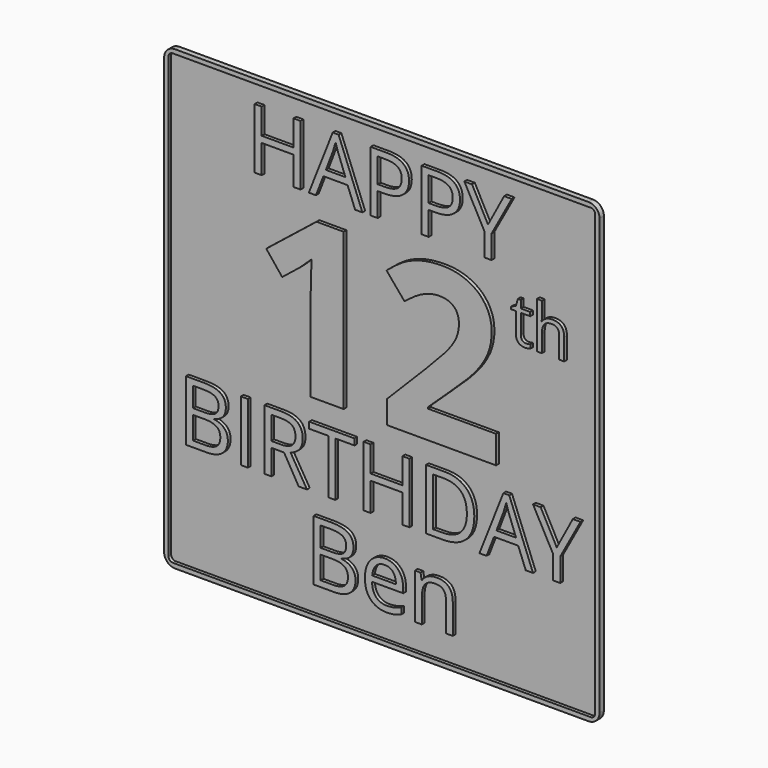
from build123d import *

# Parameters (mm, degrees)
F1_DEPTH       = 0.6
F2_TEXT_SIZE   = 24.6944444444
F2_TEXT_SIZE_2 = 63.7886434631
F2_TEXT_SIZE_3 = 17.7540454186
F3_DEPTH       = 1
F5_DEPTH       = 0.9906


# Not quite as in the source:
# - Text() gives the source's letters only with a copy of the font that has no kerning and outlines rounded to 1/6400 em; it was checked with that copy


with BuildPart() as f1:
    # F0 (on Front) → F1 (new body)
    with BuildSketch(Plane.XZ):
        with BuildLine():
            Line((123.825, 0), (3.175, 0))
            ThreePointArc((3.175, 0), (0.9299359697, -0.9299359697), (0, -3.175))
            Line((0, -3.175), (0, -130.175))
            ThreePointArc((0, -130.175), (0.9299359697, -132.4200640303), (3.175, -133.35))
            Line((3.175, -133.35), (123.825, -133.35))
            ThreePointArc((123.825, -133.35), (126.0700640303, -132.4200640303), (127, -130.175))
            Line((127, -130.175), (127, -3.175))
            ThreePointArc((127, -3.175), (126.0700640303, -0.9299359697), (123.825, 0))
        make_face()
    extrude(amount=F1_DEPTH)

    # F2 (on face) → F3 (join)
    with BuildSketch(Plane.XZ.offset(0.6)):
        with Locations((23.9946766493, -24.13)):
            Text('HAPPY', F2_TEXT_SIZE, font='Open Sans', text_align=(TextAlign.LEFT, TextAlign.BOTTOM))
        with Locations((3.9535915799, -100.5378232934)):
            Text('BIRTHDAY', F2_TEXT_SIZE, font='Open Sans', text_align=(TextAlign.LEFT, TextAlign.BOTTOM))
        with Locations((26.034138941, -76.4078232934)):
            Text('12', F2_TEXT_SIZE_2, font='Open Sans', font_style=FontStyle.BOLD, text_align=(TextAlign.LEFT, TextAlign.BOTTOM))
        with Locations((100.965861059, -43.2629127014)):
            Text('th', F2_TEXT_SIZE_3, font='Open Sans', text_align=(TextAlign.LEFT, TextAlign.BOTTOM))
        with Locations((41.1862543403, -124.3073880959)):
            Text('Ben', F2_TEXT_SIZE, font='Open Sans', text_align=(TextAlign.LEFT, TextAlign.BOTTOM))
    extrude(amount=F3_DEPTH)

    # F4 (on face) → F5 (join)
    with BuildSketch(Plane.XZ.offset(0.6)):
        with BuildLine():
            Line((127, -130.175), (127, -3.175))
            ThreePointArc((127, -3.175), (126.0700640303, -0.9299359697), (123.825, 0))
            Line((123.825, 0), (3.175, 0))
            ThreePointArc((3.175, 0), (0.9299359697, -0.9299359697), (0, -3.175))
            Line((0, -3.175), (0, -130.175))
            ThreePointArc((0, -130.175), (0.9299359697, -132.4200640303), (3.175, -133.35))
            Line((3.175, -133.35), (123.825, -133.35))
            ThreePointArc((123.825, -133.35), (126.0700640303, -132.4200640303), (127, -130.175))
        make_face()
        with BuildLine():
            ThreePointArc((1.27, -2.54), (1.6419743879, -1.6419743879), (2.54, -1.27))
            Line((2.54, -1.27), (124.46, -1.27))
            ThreePointArc((124.46, -1.27), (125.3580256121, -1.6419743879), (125.73, -2.54))
            Line((125.73, -2.54), (125.73, -130.81))
            ThreePointArc((125.73, -130.81), (125.3580256121, -131.7080256121), (124.46, -132.08))
            Line((124.46, -132.08), (2.54, -132.08))
            ThreePointArc((2.54, -132.08), (1.6419743879, -131.7080256121), (1.27, -130.81))
            Line((1.27, -130.81), (1.27, -2.54))
        make_face(mode=Mode.SUBTRACT)
    extrude(amount=F5_DEPTH)


solid = f1.part
